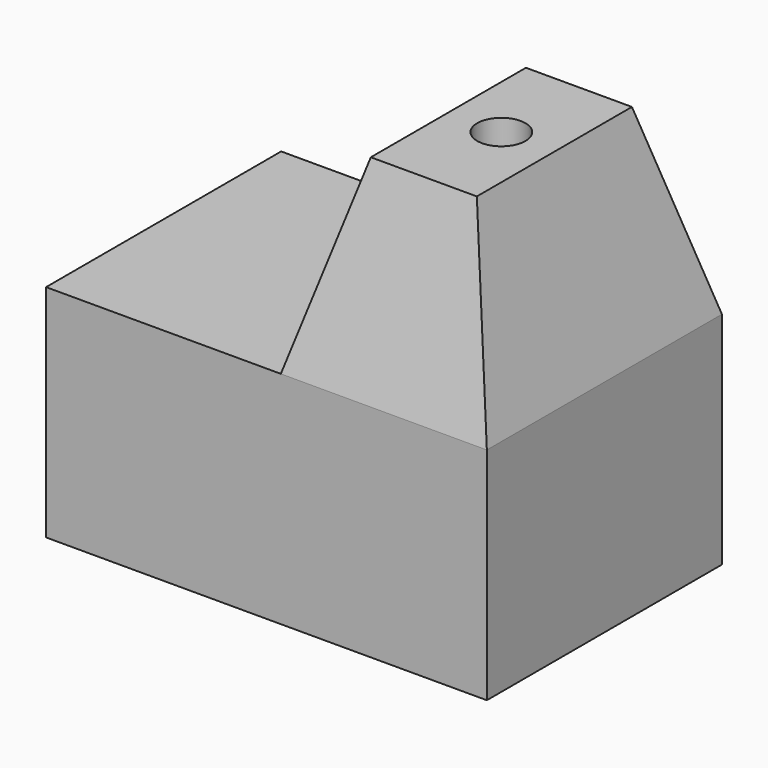
from build123d import *

# Parameters (mm, degrees)
F0_W     = 60
F0_H     = 30
F1_DEPTH = 40
F2_W     = 28.0448670685
F2_H     = 40
F3_DEPTH = 25.4
F3_TAPER = 15
F4_R     = 3.2869844705
F5_DEPTH = 25


# Not quite as in the source:
# - a feature names something its author has since deleted; it is built from what else it names


with BuildPart() as f1:
    # F0 (on Front) → F1 (new body)
    with BuildSketch(Plane.XZ):
        with Locations((-1.9551329315, 8.1626253676)):
            Rectangle(F0_W, F0_H)
    extrude(amount=F1_DEPTH)

    # F2 (on face) → F3 (join)
    with BuildSketch(Plane.XY.offset(23.1626253676)):
        with Locations((14.0224335343, -20)):
            Rectangle(F2_W, F2_H)
    extrude(amount=F3_DEPTH, taper=F3_TAPER)

    # F4 (on face) → F5 (cut)
    with BuildSketch(Plane.XY.offset(48.5626253676)):
        with Locations((14.0224335343, -20)):
            Circle(F4_R)
    extrude(amount=-F5_DEPTH, mode=Mode.SUBTRACT)


solid = f1.part
